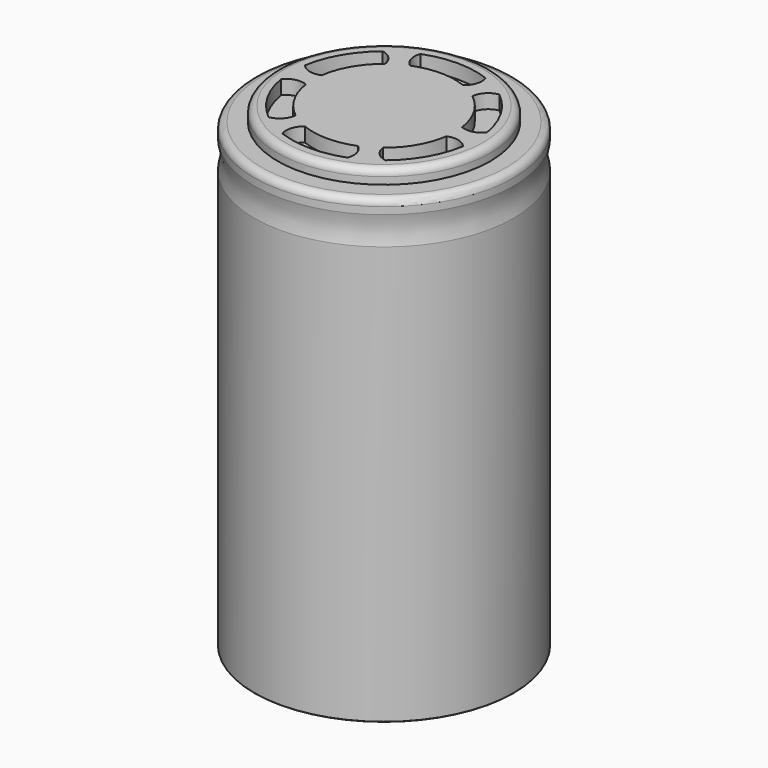
from build123d import *

# Parameters (mm, degrees)
F4_DEPTH = 2


# Not quite as in the source:
# - a feature of the source that left no trace in its solid (it failed there, or was rolled back) is left out


with BuildPart() as f2:
    # F1 (on Front) → F2 (revolve)
    with BuildSketch(Plane.XZ):
        with BuildLine():
            Line((0, 67), (0, 65))
            Line((0, 65), (15, 65))
            Line((15, 65), (15, 66))
            ThreePointArc((15, 66), (14.7071067812, 66.7071067812), (14, 67))
            Line((14, 67), (0, 67))
        make_face()
        with BuildLine():
            Line((0, 65), (0, 0))
            Line((0, 0), (18.2, 0))
            ThreePointArc((18.2, 0), (18.2707106781, 0.0292893219), (18.3, 0.1))
            Line((18.3, 0.1), (18.3, 59))
            ThreePointArc((18.3, 59), (17.9754446797, 61), (18.3, 63))
            Line((18.3, 63), (18.3, 64))
            ThreePointArc((18.3, 64), (18.0071067812, 64.7071067812), (17.3, 65))
            Line((17.3, 65), (15, 65))
            Line((15, 65), (0, 65))
        make_face()
    revolve(axis=Axis((0, 0, 33.5), (0, 0, 1)))

    # F3 (on face) → F4 (cut)
    with BuildSketch(Plane.XY.offset(67)):
        with BuildLine():
            ThreePointArc((-6.1588027163, 7.8783976227), (-6.8349323024, 9.3151975073), (-8.240042652, 10.0549339676))
            ThreePointArc((-8.240042652, 10.0549339676), (-11.2583302492, 6.5), (-12.8278495753, 2.1086192811))
            ThreePointArc((-12.8278495753, 2.1086192811), (-11.4846638338, 1.2616262534), (-9.9022938405, 1.3944807979))
            ThreePointArc((-9.9022938405, 1.3944807979), (-8.6602540378, 5), (-6.1588027163, 7.8783976227))
        make_face()
        with BuildLine():
            ThreePointArc((-3.7434911242, 9.2728784206), (0, 10), (3.7434911242, 9.2728784206))
            ThreePointArc((3.7434911242, 9.2728784206), (4.6497315314, 10.5768237606), (4.5878069233, 12.1635532487))
            ThreePointArc((4.5878069233, 12.1635532487), (0, 13), (-4.5878069233, 12.1635532487))
            ThreePointArc((-4.5878069233, 12.1635532487), (-4.6497315314, 10.5768237606), (-3.7434911242, 9.2728784206))
        make_face()
        with BuildLine():
            ThreePointArc((-9.9022938405, -1.3944807979), (-11.4846638338, -1.2616262534), (-12.8278495753, -2.1086192811))
            ThreePointArc((-12.8278495753, -2.1086192811), (-11.2583302492, -6.5), (-8.240042652, -10.0549339676))
            ThreePointArc((-8.240042652, -10.0549339676), (-6.8349323024, -9.3151975073), (-6.1588027163, -7.8783976227))
            ThreePointArc((-6.1588027163, -7.8783976227), (-8.6602540378, -5), (-9.9022938405, -1.3944807979))
        make_face()
        with BuildLine():
            ThreePointArc((-3.7434911242, -9.2728784206), (-4.6497315314, -10.5768237606), (-4.5878069233, -12.1635532487))
            ThreePointArc((-4.5878069233, -12.1635532487), (0, -13), (4.5878069233, -12.1635532487))
            ThreePointArc((4.5878069233, -12.1635532487), (4.6497315314, -10.5768237606), (3.7434911242, -9.2728784206))
            ThreePointArc((3.7434911242, -9.2728784206), (0, -10), (-3.7434911242, -9.2728784206))
        make_face()
        with BuildLine():
            ThreePointArc((6.1588027163, -7.8783976227), (6.8349323024, -9.3151975073), (8.240042652, -10.0549339676))
            ThreePointArc((8.240042652, -10.0549339676), (11.2583302492, -6.5), (12.8278495753, -2.1086192811))
            ThreePointArc((12.8278495753, -2.1086192811), (11.4846638338, -1.2616262534), (9.9022938405, -1.3944807979))
            ThreePointArc((9.9022938405, -1.3944807979), (8.6602540378, -5), (6.1588027163, -7.8783976227))
        make_face()
        with BuildLine():
            ThreePointArc((9.9022938405, 1.3944807979), (11.4846638338, 1.2616262534), (12.8278495753, 2.1086192811))
            ThreePointArc((12.8278495753, 2.1086192811), (11.2583302492, 6.5), (8.240042652, 10.0549339676))
            ThreePointArc((8.240042652, 10.0549339676), (6.8349323024, 9.3151975073), (6.1588027163, 7.8783976227))
            ThreePointArc((6.1588027163, 7.8783976227), (8.6602540378, 5), (9.9022938405, 1.3944807979))
        make_face()
    extrude(amount=-F4_DEPTH, mode=Mode.SUBTRACT)


solid = f2.part
